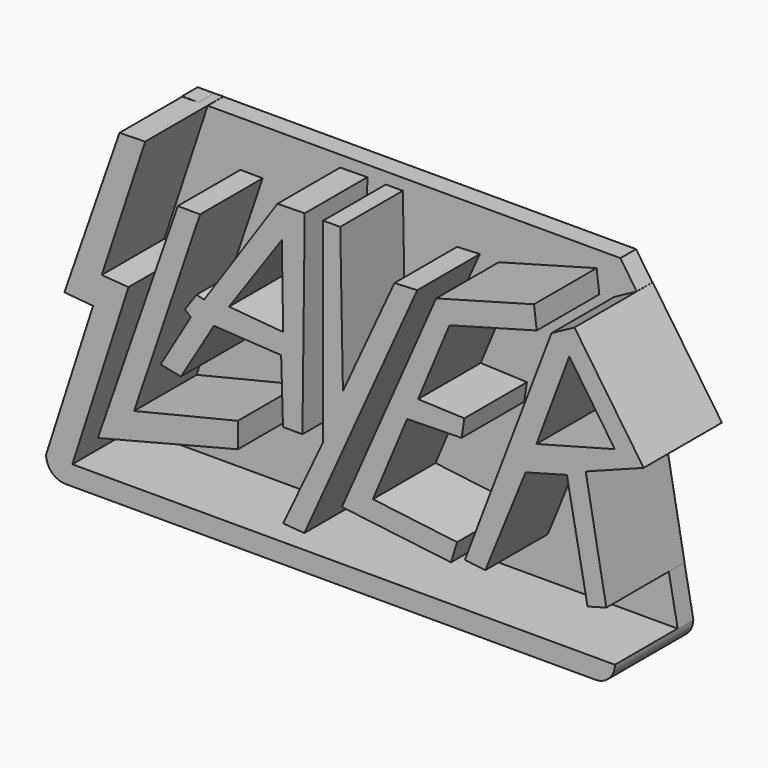
from build123d import *

# Parameters (mm, degrees)
F1_DEPTH = 25
F2_W     = 145.3895270824
F2_H     = 25
F3_DEPTH = 5
F5_DEPTH = 5
F6_R     = 4.99999


# Not quite as in the source:
# - a fillet or chamfer is up to 0.001 mm smaller than in the source, because OpenCascade refuses the exact size


with BuildPart() as f1:
    # F0 (on Front) → F1 (new body)
    with BuildSketch(Plane.XZ):
        Polygon((-49.8568192124, 39.1075946391), (-56.4118437469, 38.9586128294), (-70.5003495435, -1.5205583768), (-63.176676631, -2.1846769378), (-75.1830488443, -39.5527109504), (-68.4790462255, -39.5527109504), (-54.1241802275, 4.9719237722), (-60.960277915, 5.4854331538), align=None)
    extrude(amount=F1_DEPTH)

    # F2 (on face) → F3 (join)
    with BuildSketch(Plane(origin=(0, 0, -39.5527109504), x_dir=(1, 0, 0), z_dir=(0, 0, -1))):
        with Locations((-2.4882853031, 12.5)):
            Rectangle(F2_W, F2_H)
    extrude(amount=F3_DEPTH)

    # F6 (radius 5 in the source; OpenCascade refuses exactly that, so slightly less here)
    f6_edges = [f1.edges().sort_by_distance(p)[0] for p in [
        (70.206478, -12.5, -44.552711),
        (-75.183049, -12.5, -44.552711),
    ]]
    fillet(f6_edges, radius=F6_R)


with BuildPart() as f1b:
    # F0 (on Front) → F1, piece 2 (new body)
    with BuildSketch(Plane.XZ):
        Polygon((-52.687395364, -22.4202554673), (-35.8314104378, 27.2812079638), (-41.5140576661, 27.3383427411), (-61.9532987475, -31.5132625401), (-26.1693410575, -22.4202554673), (-26.1693410575, -16.0142090172), align=None)
    extrude(amount=F1_DEPTH)


with BuildPart() as f1c:
    # F0 (on Front) → F1, piece 3 (new body)
    with BuildSketch(Plane.XZ):
        Polygon((-9.0740518644, 36.2361818552), (-16.0388462245, 36.1280366778), (-34.8100550473, 8.4181567654), (-36.6958837116, 8.9390994981), (-39.6980270743, 4.6696574427), (-38.1983165081, 3.3758431673), (-45.9069944918, -9.7606536001), (-40.7042652369, -10.7657248154), (-32.274659742, 3.3758431673), (-15.1044856757, 2.3593353108), (-14.6315097809, -13.66269961), (-9.6652712673, -13.66269961), align=None)
        Polygon((-14.9480281398, 28.2920897007), (-14.5817017183, 7.7237756923), (-28.4223798662, 8.9390994981), align=None, mode=Mode.SUBTRACT)
    extrude(amount=F1_DEPTH)


with BuildPart() as f1d:
    # F0 (on Front) → F1, piece 4 (new body)
    with BuildSketch(Plane.XZ):
        Polygon((0, 36.1379608512), (-4.3442999013, 36.1280366778), (-4.3442999013, -13.66269961), (-14.5799871534, -35.3235378861), (-9.1679766774, -35.7429459691), (19.6837689728, 28.2920897007), (13.8670681044, 28.0186552554), (0.6849662168, -0.5772078293), align=None)
    extrude(amount=F1_DEPTH)


with BuildPart() as f1e:
    # F0 (on Front) → F1, piece 5 (new body)
    with BuildSketch(Plane.XZ):
        Polygon((50.2130747932, 29.1436510876), (49.5194196701, 34.8208174109), (24.5116390288, 28.0186552554), (0.4405695072, -26.747237891), (28.2942693621, -30.153506403), (29.8667065799, -25.0938124955), (8.352403529, -22.4202554673), (17.101412639, -1.5205583768), (31.0057803671, -1.2611554515), (31.722612679, 3.3758431673), (19.8963228613, 3.847383894), (27.9255900532, 23.0814144015), align=None)
    extrude(amount=F1_DEPTH)


with BuildPart() as f1f:
    # F0 (on Front) → F1, piece 6 (new body)
    with BuildSketch(Plane.XZ):
        Polygon((59.8610974848, 32.9642109573), (53.9944581687, 29.7904536128), (31.8534656095, -28.4306296104), (37.0677597821, -29.0682930499), (47.3705790937, -3.7012356333), (57.9263914569, -0.8300353294), (63.2158815861, -28.7272930145), (68.0079700506, -27.4238361718), (62.7463310957, 1.5151726548), (77.5532349944, 7.1303225122), align=None)
        Polygon((50.1446537673, 3.5999426618), (58.5438013077, 26.0186325759), (70.1747397517, 8.9390994981), align=None, mode=Mode.SUBTRACT)
    extrude(amount=F1_DEPTH)


with BuildPart() as f5:
    # F4 (on Front) → F5 (new body)
    with BuildSketch(Plane.XZ):
        Polygon((-62.827283707, -1.7116093077), (-75.1262456179, -39.5546890795), (70.2679157257, -39.6652817726), (62.5108405948, 1.6957151238), (77.1726742387, 7.2090495378), (55.6068457663, 39.0533618629), (-56.435116975, 39.0533618629), (-70.547408027, -1.7116093077), align=None)
    extrude(amount=F5_DEPTH)


solid = Compound([f1.part, f1b.part, f1c.part, f1d.part, f1e.part, f1f.part, f5.part])
